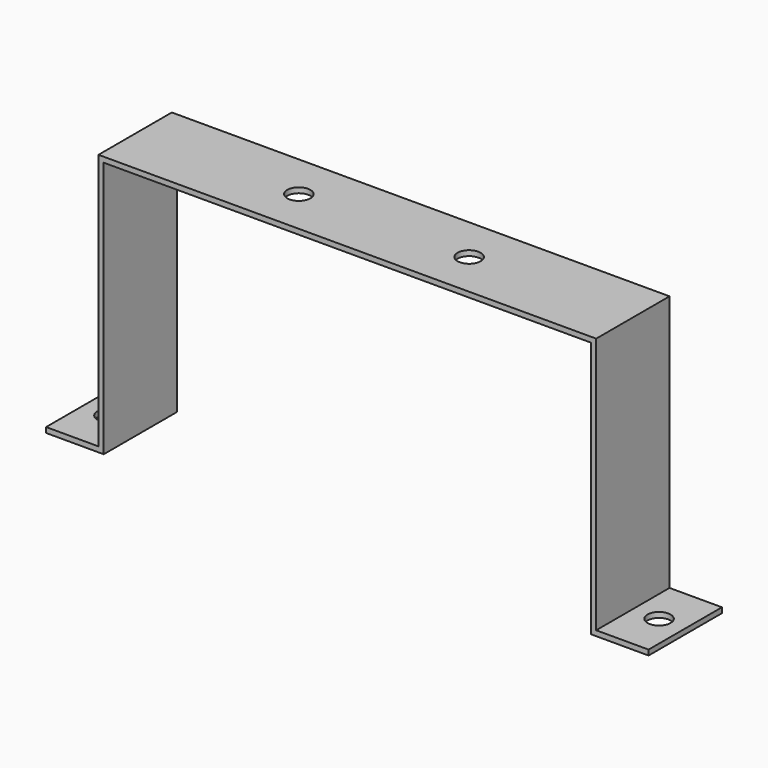
from build123d import *

# Parameters (mm, degrees)
F1_DEPTH = 17.5
F2_R     = 4.4
F3_DEPTH = 25
F4_R     = 4.4
F5_DEPTH = 25


# Not quite as in the source:
# - a feature names something its author has since deleted; it is built from what else it names


with BuildPart() as f1:
    # F0 (on Front) → F1 (new body, symmetric)
    with BuildSketch(Plane.XZ):
        Polygon((95, -38), (95, 60), (-95, 60), (-95, -38), (-115, -38), (-115, -40), (-93, -40), (-93, 58), (93, 58), (93, -40), (115, -40), (115, -38), align=None)
    extrude(amount=F1_DEPTH, both=True)

    # F2 (on face) → F3 (cut)
    with BuildSketch(Plane.XY.offset(-38)):
        with Locations((-105, 0)):
            Circle(F2_R)
        with Locations((105, 0)):
            Circle(F2_R)
    extrude(amount=-F3_DEPTH, mode=Mode.SUBTRACT)

    # F4 (on face) → F5 (cut)
    with BuildSketch(Plane.XY.offset(60)):
        with Locations((-32.5, 0)):
            Circle(F4_R)
        with Locations((32.5, 0)):
            Circle(F4_R)
    extrude(amount=-F5_DEPTH, mode=Mode.SUBTRACT)


solid = f1.part
